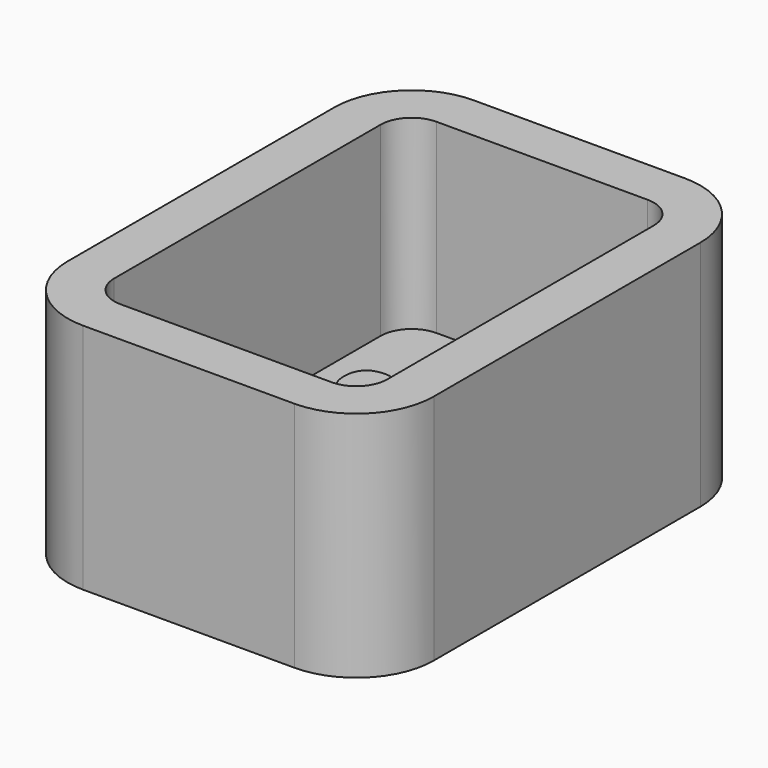
from build123d import *

# Parameters (mm, degrees)
F1_DEPTH     = 38.1
F2_T         = -7.62
F3_TEXT_SIZE = 44.0972222222
F4_DEPTH     = 5.08


# Not quite as in the source:
# - Text() gives the source's letters only with a copy of the font that has no kerning and outlines rounded to 1/6400 em; it was checked with that copy


with BuildPart() as f1:
    # F0 (on Top) → F1 (new body)
    with BuildSketch(Plane.XY):
        with BuildLine():
            ThreePointArc((30, 47.3), (26.2802561211, 56.2802561211), (17.3, 60))
            Line((17.3, 60), (-17.3, 60))
            ThreePointArc((-17.3, 60), (-26.2802561211, 56.2802561211), (-30, 47.3))
            Line((-30, 47.3), (-30, -7.3))
            ThreePointArc((-30, -7.3), (-26.2802561211, -16.2802561211), (-17.3, -20))
            Line((-17.3, -20), (17.3, -20))
            ThreePointArc((17.3, -20), (26.2802561211, -16.2802561211), (30, -7.3))
            Line((30, -7.3), (30, 47.3))
        make_face()
    extrude(amount=F1_DEPTH)

    # F2
    f2_openings = [f1.faces().sort_by_distance(p)[0] for p in [
        (0, 20, 38.1),
    ]]
    offset(amount=F2_T, openings=f2_openings)

    # F3 (on face) → F4 (join)
    with BuildSketch(Plane.XY.offset(7.62)):
        with Locations(Location((-12.3848658266, 34.3074815538), (0, 0, -90))):
            Text(':)', F3_TEXT_SIZE, font='Open Sans', font_style=FontStyle.BOLD, text_align=(TextAlign.LEFT, TextAlign.BOTTOM))
    extrude(amount=F4_DEPTH)


solid = f1.part
